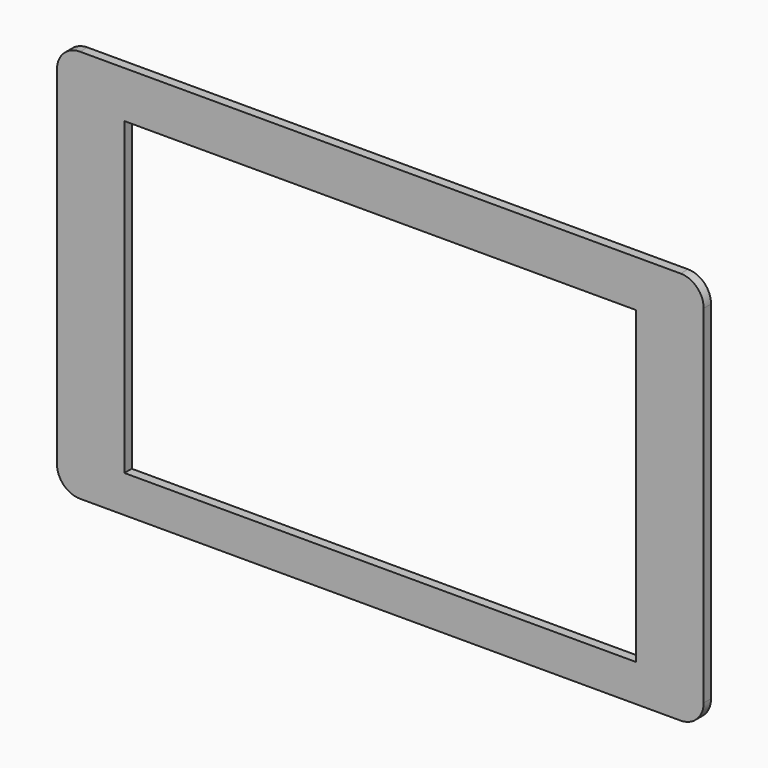
from build123d import *

# Parameters (mm, degrees)
F0_W     = 166.2
F0_H     = 100.6
F1_DEPTH = 3


# Not quite as in the source:
# - a feature names something its author has since deleted; it is built from what else it names


with BuildPart() as f1:
    # F0 (on Front) → F1 (new body)
    with BuildSketch(Plane.XZ):
        with BuildLine():
            ThreePointArc((105, 56.4), (102.8033008589, 61.7033008589), (97.5, 63.9))
            Line((97.5, 63.9), (-97.5, 63.9))
            ThreePointArc((-97.5, 63.9), (-102.8033008589, 61.7033008589), (-105, 56.4))
            Line((-105, 56.4), (-105, -56.4))
            ThreePointArc((-105, -56.4), (-102.8033008589, -61.7033008589), (-97.5, -63.9))
            Line((-97.5, -63.9), (97.5, -63.9))
            ThreePointArc((97.5, -63.9), (102.8033008589, -61.7033008589), (105, -56.4))
            Line((105, -56.4), (105, 56.4))
        make_face()
        with Locations((0, -1.55)):
            Rectangle(F0_W, F0_H, mode=Mode.SUBTRACT)
    extrude(amount=F1_DEPTH)


solid = f1.part
